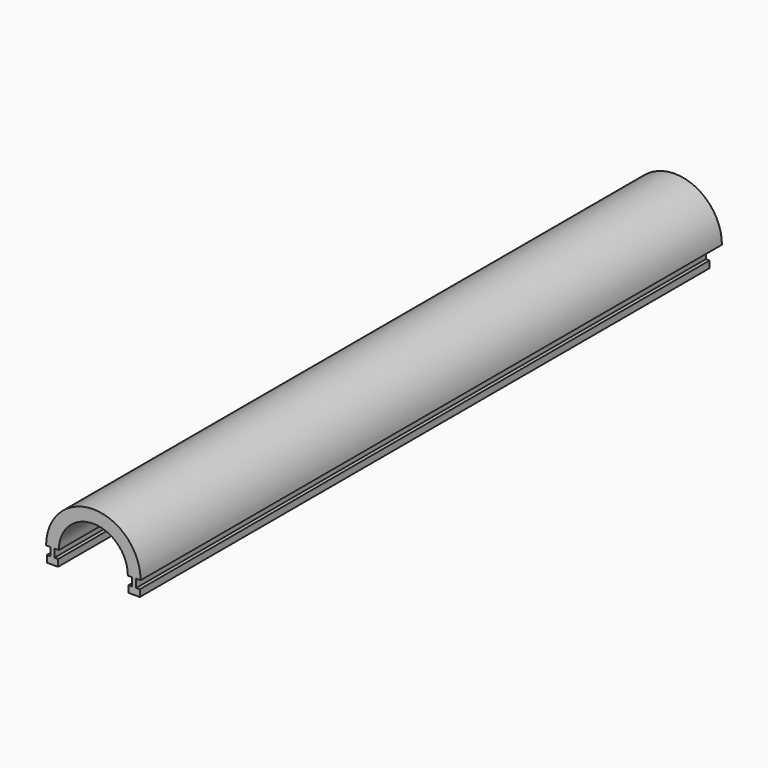
from build123d import *

# Parameters (mm, degrees)
F1_DEPTH = 63.5
F3_DEPTH = 124.46


# Not quite as in the source:
# - a pattern or mirror of a feature is missing from the dataset's text; its kind, count and spacing are read off the source's solid


with BuildPart() as f1:
    # F0 (on Front) → F1 (new body, symmetric)
    with BuildSketch(Plane.XZ):
        with BuildLine():
            ThreePointArc((-6.0325, 0), (0, 6.0325), (6.0325, 0))
            Line((6.0325, 0), (8.255, 0))
            ThreePointArc((8.255, 0), (0, 8.255), (-8.255, 0))
            Line((-8.255, 0), (-6.0325, 0))
        make_face()
    extrude(amount=F1_DEPTH, both=True)

    # F2 (on face) → F3 (join)
    with BuildSketch(Plane.XZ.offset(63.5)):
        Polygon((-6.7945, 0), (-7.493, 0), (-7.493, -1.4224), (-8.128, -1.4224), (-8.128, -2.6162), (-6.1595, -2.6162), (-6.1595, -1.4224), (-6.7945, -1.4224), align=None)
    f3 = extrude(amount=-F3_DEPTH)

    # F3_copies: F3 across plane
    add(f3.mirror(Plane(origin=(0, 0, 0), x_dir=(0, 0, 1), z_dir=(1, 0, 0))))


solid = f1.part
